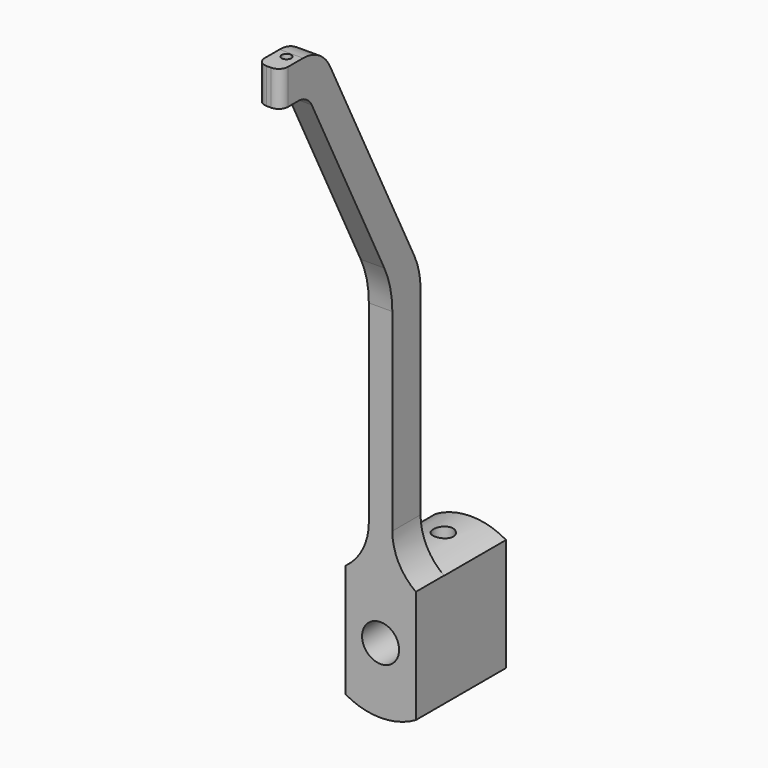
from build123d import *

# Parameters (mm, degrees)
F2_DEPTH      = 1.5875
F2_DEPTH_BACK = 1.5875
F3_DEPTH      = 9.525
F3_DEPTH_BACK = 9.525
F4_T1_DEPTH   = 62.865
F4_T6_DEPTH   = 62.865
F4_T11_DEPTH  = 62.865
F4_T16_DEPTH  = 62.865
F4_T21_DEPTH  = 62.865
F5_R          = 2.5
F6_DEPTH      = 34.1227081721
F7_R          = 1.3462
F8_DEPTH      = 25.4
F9_R          = 7.62
F10_R         = 0.635
F11_DEPTH     = 25.4
F12_R         = 1.27
F14_DEPTH     = 34.1227081721


# Not quite as in the source:
# - a fillet or chamfer that OpenCascade refuses, or shapes differently, is made with other operations: its cross-section is extruded or revolved along the edge and cut away or added
# - a feature names something its author has since deleted; it is built from what else it names


with BuildPart() as f2:
    # F1 (on Right) → F2 (new body, two sides)
    with BuildSketch(Plane.YZ) as f2_sk:
        with BuildLine():
            Line((-18.8817081721, 76.2), (-18.8817081721, 71.4375))
            Line((-18.8817081721, 71.4375), (-15.875, 71.4375))
            ThreePointArc((-15.875, 71.4375), (-14.541737999, 71.0594464463), (-13.6053613819, 70.0378247534))
            Line((-13.6053613819, 70.0378247534), (-1.35700712, 45.6593854024))
            ThreePointArc((-1.35700712, 45.6593854024), (-0.3438898526, 42.8769409358), (0, 39.9358282931))
            Line((0, 39.9358282931), (0, 8.89))
            Line((0, 8.89), (4.7625, 8.89))
            Line((4.7625, 8.89), (4.7625, 40.6322548497))
            ThreePointArc((4.7625, 40.6322548497), (4.4978433834, 42.8957264678), (3.7181513215, 45.0370875254))
            Line((3.7181513215, 45.0370875254), (-10.5324309359, 73.4006495068))
            ThreePointArc((-10.5324309359, 73.4006495068), (-12.4051841702, 75.4438928927), (-15.0717081721, 76.2))
            Line((-15.0717081721, 76.2), (-18.8817081721, 76.2))
        make_face()
    extrude(amount=F2_DEPTH)
    extrude(f2_sk.sketch, amount=-F2_DEPTH_BACK)

    # F1 (on Right) → F3 (join, two sides)
    with BuildSketch(Plane.YZ) as f3_sk:
        Polygon((4.7625, 8.89), (0, 8.89), (0, -8.89), (15.24, -8.89), (15.24, 8.89), align=None)
    extrude(amount=F3_DEPTH)
    extrude(f3_sk.sketch, amount=-F3_DEPTH_BACK)

    # F4: fillet of radius 9.525 on 4 edges, made by hand

    # F4_s2 → F4_t1 (cut)
    with BuildSketch(Plane.XZ.offset(-39.0525)):
        with BuildLine():
            ThreePointArc((9.525, 0.635), (6.7351920908, -6.1001920908), (0, -8.89))
            Line((0, -8.89), (9.525, -8.89))
            Line((9.525, -8.89), (9.525, 0.635))
        make_face()
        with BuildLine():
            ThreePointArc((-9.525, 0.635), (-6.7351920908, -6.1001920908), (0, -8.89))
            Line((0, -8.89), (-9.525, -8.89))
            Line((-9.525, -8.89), (-9.525, 0.635))
        make_face()
    extrude(amount=F4_T1_DEPTH, mode=Mode.SUBTRACT)


with BuildPart() as f4_tool4:
    # F4_s5 → F4_t6 (new body)
    with BuildSketch(Plane.XZ.offset(23.8125)):
        with BuildLine():
            ThreePointArc((0, 8.89), (6.7351920908, 6.1001920908), (9.525, -0.635))
            Line((9.525, -0.635), (9.525, 8.89))
            Line((9.525, 8.89), (0, 8.89))
        make_face()
    extrude(amount=-F4_T6_DEPTH)

    split(bisect_by=Plane.YZ.offset(1.5875), keep=Keep.TOP)


with BuildPart() as f2_1:
    add(f2.part)

    # F4_t3: cut F4_tool4
    add(f4_tool4.part, mode=Mode.SUBTRACT)


with BuildPart() as f4_tool9:
    # F4_s10 → F4_t11 (new body)
    with BuildSketch(Plane.XZ.offset(23.8125)):
        with BuildLine():
            ThreePointArc((0, 8.89), (6.7351920908, 6.1001920908), (9.525, -0.635))
            Line((9.525, -0.635), (9.525, 8.89))
            Line((9.525, 8.89), (0, 8.89))
        make_face()
    extrude(amount=-F4_T11_DEPTH)

    split(bisect_by=Plane.XZ.offset(-4.7625), keep=Keep.BOTTOM)


with BuildPart() as f2_2:
    add(f2_1.part)

    # F4_t8: cut F4_tool9
    add(f4_tool9.part, mode=Mode.SUBTRACT)


with BuildPart() as f4_tool14:
    # F4_s15 → F4_t16 (new body)
    with BuildSketch(Plane.XZ.offset(-39.0525)):
        with BuildLine():
            ThreePointArc((0, 8.89), (-6.7351920908, 6.1001920908), (-9.525, -0.635))
            Line((-9.525, -0.635), (-9.525, 8.89))
            Line((-9.525, 8.89), (0, 8.89))
        make_face()
    extrude(amount=F4_T16_DEPTH)

    split(bisect_by=Plane.XZ.offset(-4.7625), keep=Keep.BOTTOM)


with BuildPart() as f2_3:
    add(f2_2.part)

    # F4_t13: cut F4_tool14
    add(f4_tool14.part, mode=Mode.SUBTRACT)


with BuildPart() as f4_tool19:
    # F4_s20 → F4_t21 (new body)
    with BuildSketch(Plane.XZ.offset(-39.0525)):
        with BuildLine():
            ThreePointArc((0, 8.89), (-6.7351920908, 6.1001920908), (-9.525, -0.635))
            Line((-9.525, -0.635), (-9.525, 8.89))
            Line((-9.525, 8.89), (0, 8.89))
        make_face()
    extrude(amount=F4_T21_DEPTH)

    split(bisect_by=Plane.YZ.offset(-1.5875), keep=Keep.BOTTOM)


with BuildPart() as f2_4:
    add(f2_3.part)

    # F4_t18: cut F4_tool19
    add(f4_tool19.part, mode=Mode.SUBTRACT)

    # F5 (on face) → F6 (cut, through all)
    with BuildSketch(Plane(origin=(0, 15.24, 0), x_dir=(-1, 0, 0), z_dir=(0, 1, 0))):
        Circle(F5_R)
    extrude(amount=-F6_DEPTH, mode=Mode.SUBTRACT)

    # F7 (on Top) → F8 (cut)
    with BuildSketch(Plane.XY):
        with Locations((0, 10.5804353952)):
            Circle(F7_R)
        with Locations((0, -26.9685275853)):
            Circle(F7_R)
    extrude(amount=F8_DEPTH, mode=Mode.SUBTRACT)

    # F9
    f9_edges = [f2_4.edges().sort_by_distance(p)[0] for p in [
        (-9.50381, 7.62, 0),
        (-1.5875, 2.38125, 8.756777),
        (1.5875, 2.38125, 8.756777),
    ]]
    fillet(f9_edges, radius=F9_R)

    # F10 (on face) → F11 (cut)
    with BuildSketch(Plane.XY.offset(76.2)):
        with Locations((0, -15.8845081721)):
            Circle(F10_R)
    extrude(amount=-F11_DEPTH, mode=Mode.SUBTRACT)

    # F12
    f12_edges = [f2_4.edges().sort_by_distance(p)[0] for p in [
        (1.5875, -18.881708, 73.81875),
        (-1.5875, -18.881708, 73.81875),
    ]]
    fillet(f12_edges, radius=F12_R)

    # F13 (on face) → F14 (cut, through all)
    with BuildSketch(Plane(origin=(0, 15.24, 0), x_dir=(-1, 0, 0), z_dir=(0, 1, 0))):
        Polygon((-4.7625, -11.6415646072), (-4.7625, 10.8039603039), (-9.6872693895, 10.8039603039), (-9.6872693895, -15.5402623288), (11.7396748797, -15.5402623288), (11.7396748797, 10.8039603039), (4.7625, 10.8039603039), (4.7625, -11.6415646072), align=None)
    extrude(amount=-F14_DEPTH, mode=Mode.SUBTRACT)


solid = f2_4.part
